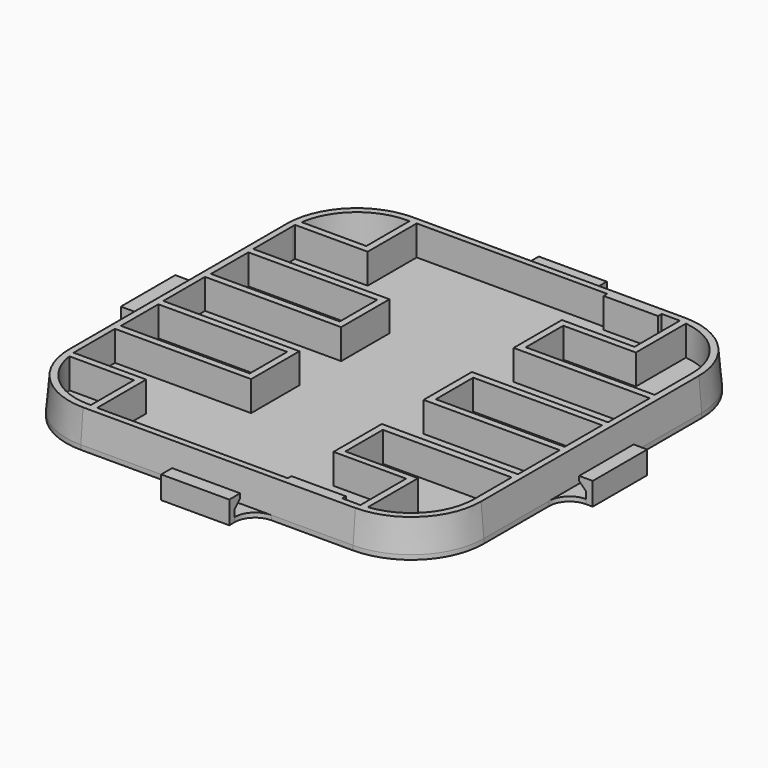
from build123d import *

# Parameters (mm, degrees)
F4_DEPTH     = 1.4
F5_W         = 30
F5_H         = 13.3
F5_W_2       = 12
F5_H_2       = 1
F6_DEPTH     = 6.6
F8_DEPTH     = 6.6
F9_W         = 14
F9_H         = 13.5
F10_DEPTH    = 6.6
F11_W        = 28.3875793553
F11_H        = 10.3
F12_DEPTH    = 6.6
F14_DEPTH    = 5.001
F15_T1_DEPTH = 1


# Not quite as in the source:
# - a fillet or chamfer that OpenCascade refuses, or shapes differently, is made with other operations: its cross-section is extruded or revolved along the edge and cut away or added


with BuildPart() as f2:
    # F2: sweep along a path in F0
    with BuildLine(Plane.XY) as f2_path:
        ThreePointArc((52, 30), (45.5563491861, 45.5563491861), (30, 52))
        Line((30, 52), (0, 52))
        Line((0, 52), (-30, 52))
        ThreePointArc((-30, 52), (-45.5563491861, 45.5563491861), (-52, 30))
        Line((-52, 30), (-52, 0))
        Line((-52, 0), (-52, -30))
        ThreePointArc((-52, -30), (-45.5563491861, -45.5563491861), (-30, -52))
        Line((-30, -52), (0, -52))
        Line((0, -52), (30, -52))
        ThreePointArc((30, -52), (45.5563491861, -45.5563491861), (52, -30))
        Line((52, -30), (52, 0))
        Line((52, 0), (52, 30))
    # F1 (on Front) → F2 (sweep)
    with BuildSketch(Plane.XZ):
        Polygon((44, 8), (44, 0), (52, 0), (52, 1), (52, 5), (49, 5), (49, 4), (50.5, 2.5), (50.5, 1), (46, 1), (45.3875793553, 8), align=None)
    sweep(path=f2_path.line)

    # F3 (on Top) → F4 (join)
    with BuildSketch(Plane.XY):
        with BuildLine():
            ThreePointArc((-44, -30), (-39.8994949366, -39.8994949366), (-30, -44))
            Line((-30, -44), (30, -44))
            ThreePointArc((30, -44), (39.8994949366, -39.8994949366), (44, -30))
            Line((44, -30), (44, 30))
            ThreePointArc((44, 30), (39.8994949366, 39.8994949366), (30, 44))
            Line((30, 44), (-30, 44))
            ThreePointArc((-30, 44), (-39.8994949366, 39.8994949366), (-44, 30))
            Line((-44, 30), (-44, -30))
        make_face()
    extrude(amount=F4_DEPTH)

    # F5 (on face) → F6 (join, through all)
    with BuildSketch(Plane.XY.offset(1.4)):
        with Locations((29, 24.85)):
            Rectangle(F5_W, F5_H)
        with Locations((20, 43.5)):
            Rectangle(F5_W_2, F5_H_2)
        with Locations((29, 0.05)):
            Rectangle(F5_W, F5_H)
        with Locations((29, -24.75)):
            Rectangle(F5_W, F5_H)
        with Locations((20, -43.5)):
            Rectangle(F5_W_2, F5_H_2)
        with BuildLine():
            ThreePointArc((-30, 44), (-39.7211110476, 40.0747208398), (-43.9910685796, 30.5))
            Line((-43.9910685796, 30.5), (-14, 30.5))
            Line((-14, 30.5), (-14, 44))
            Line((-14, 44), (-30, 44))
        make_face()
        with BuildLine():
            Line((-43.9910685796, 30.5), (-44, 30.5))
            Line((-44, 30.5), (-44, 30))
            ThreePointArc((-44, 30), (-43.9977669668, 30.250039882), (-43.9910685796, 30.5))
        make_face()
        with BuildLine():
            Line((-44, -30.5), (-43.9910685796, -30.5))
            ThreePointArc((-43.9910685796, -30.5), (-43.9977669668, -30.250039882), (-44, -30))
            Line((-44, -30), (-44, -30.5))
        make_face()
        with BuildLine():
            Line((-30, -44), (-14, -44))
            Line((-14, -44), (-14, -30.5))
            Line((-14, -30.5), (-43.9910685796, -30.5))
            ThreePointArc((-43.9910685796, -30.5), (-39.7211110476, -40.0747208398), (-30, -44))
        make_face()
        with Locations((-29, 12.35)):
            Rectangle(F5_W, F5_H)
        with Locations((-29, -12.45)):
            Rectangle(F5_W, F5_H)
    extrude(amount=F6_DEPTH)

    # F7 (on face) → F8 (join, through all)
    with BuildSketch(Plane.XY.offset(1.4)):
        with BuildLine():
            Line((43.9298241195, -31.4), (30, -31.4))
            Line((30, -31.4), (30, -44))
            ThreePointArc((30, -44), (39.3914855055, -40.3826778819), (43.9298241195, -31.4))
        make_face()
        with BuildLine():
            ThreePointArc((43.9194109071, 31.5), (39.3541434669, 40.416333328), (30, 44))
            Line((30, 44), (30, 31.5))
            Line((30, 31.5), (43.9194109071, 31.5))
        make_face()
    extrude(amount=F8_DEPTH)

    # F9 (on face) → F10 (cut, through all)
    with BuildSketch(Plane.XY.offset(8)):
        with Locations((-21, 37.25)):
            Rectangle(F9_W, F9_H)
        with Locations((-21, -37.25)):
            Rectangle(F9_W, F9_H)
    extrude(amount=-F10_DEPTH, mode=Mode.SUBTRACT)

    # F11 (on face) → F12 (cut, through all)
    with BuildSketch(Plane.XY.offset(8)):
        with BuildLine():
            Line((-43.7428112244, 32), (-29.5, 32))
            Line((-29.5, 32), (-29.5, 43.8875793553))
            Line((-29.5, 43.8875793553), (-30, 43.8875793553))
            ThreePointArc((-30, 43.8875793553), (-39.0854196832, 40.5033332581), (-43.7428112244, 32))
        make_face()
        with BuildLine():
            Line((15.5, 19.6999999465), (43.8875793553, 19.6999999465))
            Line((43.8875793553, 19.6999999465), (43.8875793553, 29.9999999465))
            ThreePointArc((43.8875793553, 30), (40.3367361721, 39.274521317), (31.5, 43.8063340663))
            Line((31.5, 43.8063340663), (31.5, 29.9999999465))
            Line((31.5, 29.9999999465), (15.5, 29.9999999465))
            Line((15.5, 29.9999999465), (15.5, 19.6999999465))
        make_face()
        with Locations((29.6937896777, 0.05)):
            Rectangle(F11_W, F11_H)
        with BuildLine():
            Line((31.5, -29.9999999465), (31.5, -43.8063340663))
            ThreePointArc((31.5, -43.8063340663), (40.3367361721, -39.274521317), (43.8875793553, -30))
            Line((43.8875793553, -29.9999999465), (43.8875793553, -29.9))
            Line((43.8875793553, -29.9), (43.8875793553, -19.6999999465))
            Line((43.8875793553, -19.6999999465), (15.5, -19.6999999465))
            Line((15.5, -19.6999999465), (15.5, -29.9))
            Line((15.5, -29.9), (15.5, -29.9999999465))
            Line((15.5, -29.9999999465), (31.5, -29.9999999465))
        make_face()
        with Locations((-29.6937896777, 12.35)):
            Rectangle(F11_W, F11_H)
        with Locations((-29.6937896777, -12.45)):
            Rectangle(F11_W, F11_H)
        with BuildLine():
            Line((-29.5, -32), (-43.7428112244, -32))
            ThreePointArc((-43.7428112244, -32), (-39.0854196832, -40.5033332581), (-30, -43.8875793553))
            Line((-30, -43.8875793553), (-29.5, -43.8875793553))
            Line((-29.5, -43.8875793553), (-29.5, -32))
        make_face()
    extrude(amount=-F12_DEPTH, mode=Mode.SUBTRACT)

    # F13 (on Top) → F14 (cut, through all)
    with BuildSketch(Plane.XY):
        with BuildLine():
            Line((52, -30), (52, -7.5))
            Line((52, -7.5), (46, -7.5))
            Line((46, -7.5), (46, -30))
            ThreePointArc((46, -30), (41.313708499, -41.313708499), (30, -46))
            Line((30, -46), (7.5, -46))
            Line((7.5, -46), (7.5, -52))
            Line((7.5, -52), (30, -52))
            ThreePointArc((30, -52), (45.5563491861, -45.5563491861), (52, -30))
        make_face()
        with BuildLine():
            Line((-30, -52), (-7.5, -52))
            Line((-7.5, -52), (-7.5, -46))
            Line((-7.5, -46), (-30, -46))
            ThreePointArc((-30, -46), (-41.313708499, -41.313708499), (-46, -30))
            Line((-46, -30), (-46, -7.5))
            Line((-46, -7.5), (-52, -7.5))
            Line((-52, -7.5), (-52, -30))
            ThreePointArc((-52, -30), (-45.5563491861, -45.5563491861), (-30, -52))
        make_face()
        with BuildLine():
            Line((-7.5, 46), (-7.5, 52))
            Line((-7.5, 52), (-30, 52))
            ThreePointArc((-30, 52), (-45.5563491861, 45.5563491861), (-52, 30))
            Line((-52, 30), (-52, 7.5))
            Line((-52, 7.5), (-46, 7.5))
            Line((-46, 7.5), (-46, 30))
            ThreePointArc((-46, 30), (-41.313708499, 41.313708499), (-30, 46))
            Line((-30, 46), (-7.5, 46))
        make_face()
        with BuildLine():
            ThreePointArc((30, 46), (41.313708499, 41.313708499), (46, 30))
            Line((46, 30), (46, 7.5))
            Line((46, 7.5), (52, 7.5))
            Line((52, 7.5), (52, 30))
            ThreePointArc((52, 30), (45.5563491861, 45.5563491861), (30, 52))
            Line((30, 52), (7.5, 52))
            Line((7.5, 52), (7.5, 46))
            Line((7.5, 46), (30, 46))
        make_face()
    extrude(amount=F14_DEPTH, mode=Mode.SUBTRACT)

    # F15: fillet of radius 4.5 on 8 edges, made by hand

    # F15_s2 → F15_t1 (join)
    with BuildSketch(Plane.XY):
        with BuildLine():
            ThreePointArc((-46, 12), (-47.3180194847, 8.8180194847), (-50.5, 7.5))
            Line((-50.5, 7.5), (-46, 7.5))
            Line((-46, 7.5), (-46, 12))
        make_face()
        with BuildLine():
            ThreePointArc((-12, 46), (-8.8180194847, 47.3180194847), (-7.5, 50.5))
            Line((-7.5, 50.5), (-7.5, 46))
            Line((-7.5, 46), (-12, 46))
        make_face()
        with BuildLine():
            ThreePointArc((12, 46), (8.8180194847, 47.3180194847), (7.5, 50.5))
            Line((7.5, 50.5), (7.5, 46))
            Line((7.5, 46), (12, 46))
        make_face()
        with BuildLine():
            ThreePointArc((12, -46), (8.8180194847, -47.3180194847), (7.5, -50.5))
            Line((7.5, -50.5), (7.5, -46))
            Line((7.5, -46), (12, -46))
        make_face()
        with BuildLine():
            ThreePointArc((-12, -46), (-8.8180194847, -47.3180194847), (-7.5, -50.5))
            Line((-7.5, -50.5), (-7.5, -46))
            Line((-7.5, -46), (-12, -46))
        make_face()
        with BuildLine():
            ThreePointArc((-46, -12), (-47.3180194847, -8.8180194847), (-50.5, -7.5))
            Line((-50.5, -7.5), (-46, -7.5))
            Line((-46, -7.5), (-46, -12))
        make_face()
        with BuildLine():
            ThreePointArc((46, -12), (47.3180194847, -8.8180194847), (50.5, -7.5))
            Line((50.5, -7.5), (46, -7.5))
            Line((46, -7.5), (46, -12))
        make_face()
        with BuildLine():
            ThreePointArc((46, 12), (47.3180194847, 8.8180194847), (50.5, 7.5))
            Line((50.5, 7.5), (46, 7.5))
            Line((46, 7.5), (46, 12))
        make_face()
    extrude(amount=F15_T1_DEPTH)


solid = f2.part
